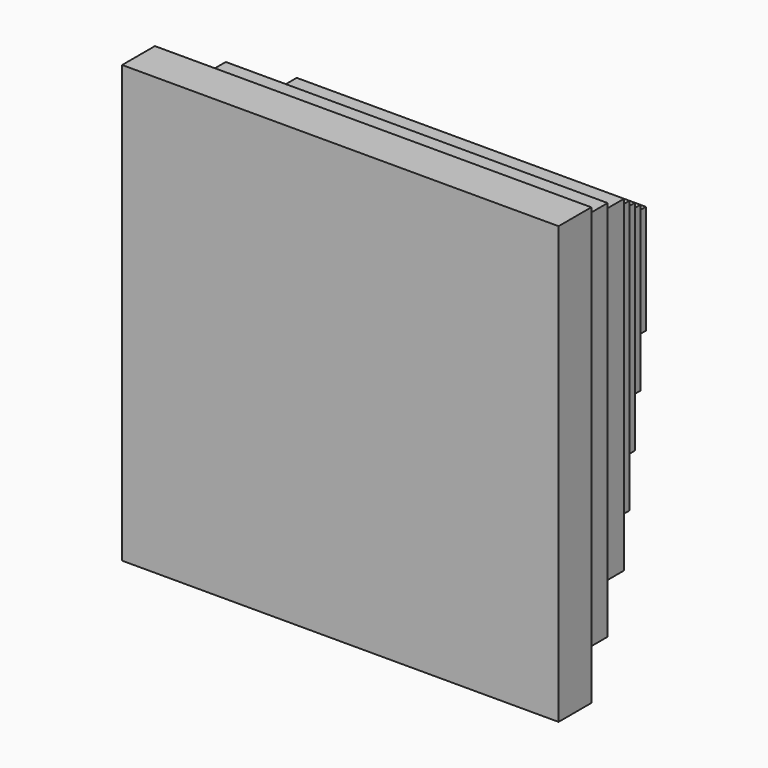
from build123d import *

# Parameters (mm, degrees)
F0_W       = 101.6
F0_H       = 101.6
F1_DEPTH   = 25.4
F2_W       = 88.9
F2_H       = 88.9
F3_DEPTH   = 25.4
F4_W       = 76.2
F4_H       = 76.2
F5_DEPTH   = 25.4
F6_W       = 63.5
F6_H       = 63.5
F7_DEPTH   = 19.05
F8_W       = 50.8
F8_H       = 50.8
F9_DEPTH   = 19.05
F10_W      = 38.1
F10_H      = 38.1
F11_DEPTH  = 19.05
F12_W      = 25.4
F12_H      = 25.4
F13_DEPTH  = 19.05
F14_SIZE   = 6.34999
F14_2_SIZE = 6.34999


# Not quite as in the source:
# - a fillet or chamfer is up to 0.001 mm smaller than in the source, because OpenCascade refuses the exact size
# - a feature names something its author has since deleted; it is built from what else it names


with BuildPart() as f1:
    # F0 (on Front) → F1 (new body)
    with BuildSketch(Plane.XZ):
        with Locations((-50.8, 50.8)):
            Rectangle(F0_W, F0_H)
        with Locations((50.8, 50.8)):
            Rectangle(F0_W, F0_H)
        with Locations((50.8, -50.8)):
            Rectangle(F0_W, F0_H)
        with Locations((-50.8, -50.8)):
            Rectangle(F0_W, F0_H)
    extrude(amount=-F1_DEPTH)

    # F2 (on face) → F3 (join)
    with BuildSketch(Plane(origin=(0, 25.4, 0), x_dir=(-1, 0, 0), z_dir=(0, 1, 0))):
        with Locations((-44.45, 44.45)):
            Rectangle(F2_W, F2_H)
        with Locations((44.45, 44.45)):
            Rectangle(F2_W, F2_H)
        with Locations((44.45, -44.45)):
            Rectangle(F2_W, F2_H)
        with Locations((-44.45, -44.45)):
            Rectangle(F2_W, F2_H)
    extrude(amount=F3_DEPTH)

    # F4 (on face) → F5 (join)
    with BuildSketch(Plane(origin=(0, 50.8, 0), x_dir=(-1, 0, 0), z_dir=(0, 1, 0))):
        with Locations((-38.1, 38.1)):
            Rectangle(F4_W, F4_H)
        with Locations((38.1, 38.1)):
            Rectangle(F4_W, F4_H)
        with Locations((38.1, -38.1)):
            Rectangle(F4_W, F4_H)
        with Locations((-38.1, -38.1)):
            Rectangle(F4_W, F4_H)
    extrude(amount=F5_DEPTH)

    # F14#2 (size 6.35 in the source; OpenCascade refuses exactly that, so slightly less here)
    f14_2_edges = [f1.edges().sort_by_distance(p)[0] for p in [
        (-76.2, 76.2, 0),
        (0, 76.2, 76.2),
        (76.2, 76.2, 0),
        (0, 76.2, -76.2),
        (-88.9, 50.8, 0),
        (0, 50.8, -88.9),
        (0, 50.8, 88.9),
        (88.9, 50.8, 0),
        (-76.2, 50.8, 0),
        (0, 50.8, 76.2),
        (76.2, 50.8, 0),
        (0, 50.8, -76.2),
        (101.6, 25.4, 0),
        (0, 25.4, -101.6),
        (0, 25.4, 101.6),
        (-101.6, 25.4, 0),
        (0, 25.4, -88.9),
        (88.9, 25.4, 0),
        (0, 25.4, 88.9),
        (-88.9, 25.4, 0),
    ]]
    chamfer(f14_2_edges, length=F14_2_SIZE)


with BuildPart() as f7:
    # F6 (on face) → F7 (new body)
    with BuildSketch(Plane(origin=(0, 76.2, 0), x_dir=(-1, 0, 0), z_dir=(0, 1, 0))):
        with Locations((31.75, 31.75)):
            Rectangle(F6_W, F6_H)
        with Locations((-31.75, 31.75)):
            Rectangle(F6_W, F6_H)
        with Locations((-31.75, -31.75)):
            Rectangle(F6_W, F6_H)
        with Locations((31.75, -31.75)):
            Rectangle(F6_W, F6_H)
    extrude(amount=F7_DEPTH)

    # F8 (on face) → F9 (join)
    with BuildSketch(Plane(origin=(0, 95.25, 0), x_dir=(-1, 0, 0), z_dir=(0, 1, 0))):
        with Locations((-25.4, -25.4)):
            Rectangle(F8_W, F8_H)
        with Locations((25.4, -25.4)):
            Rectangle(F8_W, F8_H)
        with Locations((-25.4, 25.4)):
            Rectangle(F8_W, F8_H)
        with Locations((25.4, 25.4)):
            Rectangle(F8_W, F8_H)
    extrude(amount=F9_DEPTH)

    # F10 (on face) → F11 (join)
    with BuildSketch(Plane(origin=(0, 114.3, 0), x_dir=(-1, 0, 0), z_dir=(0, 1, 0))):
        with Locations((19.05, 19.05)):
            Rectangle(F10_W, F10_H)
        with Locations((19.05, -19.05)):
            Rectangle(F10_W, F10_H)
        with Locations((-19.05, -19.05)):
            Rectangle(F10_W, F10_H)
        with Locations((-19.05, 19.05)):
            Rectangle(F10_W, F10_H)
    extrude(amount=F11_DEPTH)

    # F12 (on face) → F13 (join)
    with BuildSketch(Plane(origin=(0, 133.35, 0), x_dir=(-1, 0, 0), z_dir=(0, 1, 0))):
        with Locations((-12.7, -12.7)):
            Rectangle(F12_W, F12_H)
        with Locations((-12.7, 12.7)):
            Rectangle(F12_W, F12_H)
        with Locations((12.7, 12.7)):
            Rectangle(F12_W, F12_H)
        with Locations((12.7, -12.7)):
            Rectangle(F12_W, F12_H)
    extrude(amount=F13_DEPTH)

    # F14 (size 6.35 in the source; OpenCascade refuses exactly that, so slightly less here)
    f14_edges = [f7.edges().sort_by_distance(p)[0] for p in [
        (0, 152.4, 25.4),
        (25.4, 152.4, 0),
        (0, 152.4, -25.4),
        (-25.4, 152.4, 0),
        (0, 133.35, -38.1),
        (38.1, 133.35, 0),
        (-38.1, 133.35, 0),
        (0, 133.35, 38.1),
        (0, 133.35, 25.4),
        (25.4, 133.35, 0),
        (0, 133.35, -25.4),
        (-25.4, 133.35, 0),
        (0, 114.3, -50.8),
        (50.8, 114.3, 0),
        (-50.8, 114.3, 0),
        (0, 114.3, 50.8),
        (0, 114.3, -38.1),
        (-38.1, 114.3, 0),
        (0, 114.3, 38.1),
        (38.1, 114.3, 0),
        (0, 95.25, 63.5),
        (-63.5, 95.25, 0),
        (63.5, 95.25, 0),
        (0, 95.25, -63.5),
        (0, 95.25, -50.8),
        (-50.8, 95.25, 0),
        (0, 95.25, 50.8),
        (50.8, 95.25, 0),
    ]]
    chamfer(f14_edges, length=F14_SIZE)


solid = Compound([f1.part, f7.part])
